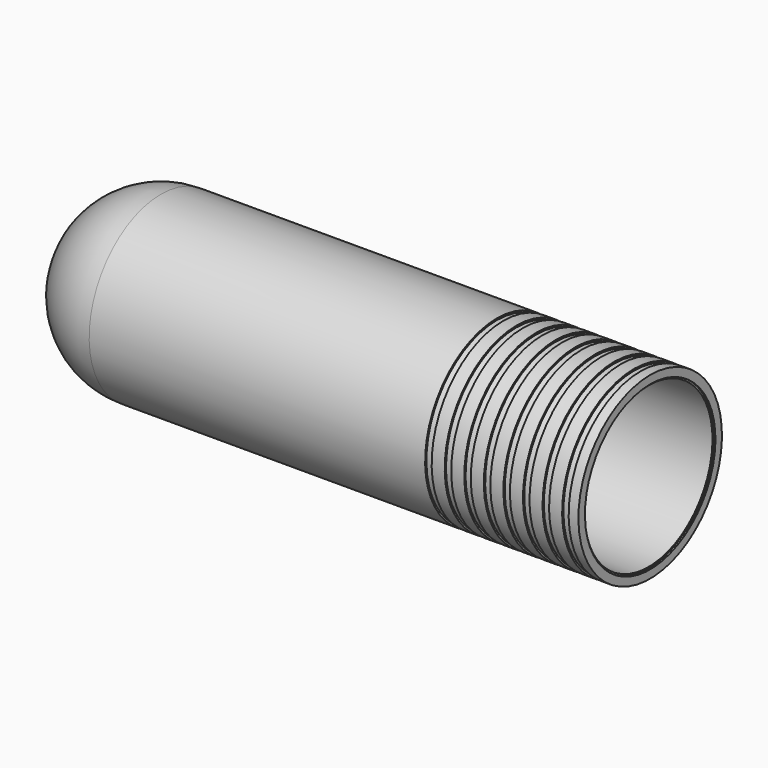
from build123d import *

# Parameters (mm, degrees)
F2_T = 2.5


# Not quite as in the source:
# - a shell that OpenCascade refuses in one call is made with other operations: the cavity is built on its own and cut out


with BuildPart() as f1:
    # F0 (on Front) → F1 (revolve)
    with BuildSketch(Plane.XZ):
        with BuildLine():
            Line((-96.4535274908, 0), (81.0464725092, 0))
            Line((81.0464725092, 0), (81.0464725092, 27.5))
            Line((81.0464725092, 27.5), (78.0464725092, 27.5))
            Line((78.0464725092, 27.5), (78.0464725092, 27))
            Line((78.0464725092, 27), (76.0464725092, 27))
            Line((76.0464725092, 27), (76.0464725092, 27.5))
            Line((76.0464725092, 27.5), (72.0464725092, 27.5))
            Line((72.0464725092, 27.5), (72.0464725092, 27))
            Line((72.0464725092, 27), (70.0464725092, 27))
            Line((70.0464725092, 27), (70.0464725092, 27.5))
            Line((70.0464725092, 27.5), (66.0464725092, 27.5))
            Line((66.0464725092, 27.5), (66.0464725092, 27))
            Line((66.0464725092, 27), (64.0464725092, 27))
            Line((64.0464725092, 27), (64.0464725092, 27.5))
            Line((64.0464725092, 27.5), (60.0464725092, 27.5))
            Line((60.0464725092, 27.5), (60.0464725092, 27))
            Line((60.0464725092, 27), (58.0464725092, 27))
            Line((58.0464725092, 27), (58.0464725092, 27.5))
            Line((58.0464725092, 27.5), (56.0464725092, 27.5))
            Line((56.0464725092, 27.5), (54.0464725092, 27.5))
            Line((54.0464725092, 27.5), (54.0464725092, 27))
            Line((54.0464725092, 27), (52.0464725092, 27))
            Line((52.0464725092, 27), (52.0464725092, 27.5))
            Line((52.0464725092, 27.5), (48.0464725092, 27.5))
            Line((48.0464725092, 27.5), (48.0464725092, 27))
            Line((48.0464725092, 27), (46.0464725092, 27))
            Line((46.0464725092, 27), (46.0464725092, 27.5))
            Line((46.0464725092, 27.5), (42.0464725092, 27.5))
            Line((42.0464725092, 27.5), (42.0464725092, 27))
            Line((42.0464725092, 27), (40.0464725092, 27))
            Line((40.0464725092, 27), (40.0464725092, 27.5))
            Line((40.0464725092, 27.5), (36.0464725092, 27.5))
            Line((36.0464725092, 27.5), (36.0464725092, 27))
            Line((36.0464725092, 27), (34.0464725092, 27))
            Line((34.0464725092, 27), (34.0464725092, 27.5))
            Line((34.0464725092, 27.5), (32.0464725092, 27.5))
            Line((32.0464725092, 27.5), (25.0464725092, 27.5))
            Line((25.0464725092, 27.5), (-68.9535274908, 27.5))
            ThreePointArc((-68.9535274908, 27.5), (-88.3989639735, 19.4454364826), (-96.4535274908, 0))
        make_face()
    revolve(axis=Axis((-7.7035274908, 0, 0), (-1, 0, 0)))

    # F2: shell of thickness 2.5, made by hand


with BuildPart() as f2_core1:
    # F2_t2: copy of F1
    add(f1.part)

    # the walls: a layer under each face that stays
    f2_faces = [f2_core1.faces().sort_by_distance(p)[0] for p in [
        (-88.3989639735, 0, -19.4454364826),
        (-17.4535274908, 0, -27.5),
        (34.0464725092, -13.2407407407, -24.0625),
        (35.0464725092, 0, -27),
        (36.0464725092, -13.2407407407, 24.0625),
        (38.0464725092, 0, -27.5),
        (40.0464725092, -13.2407407407, -24.0625),
        (41.0464725092, 0, -27),
        (42.0464725092, -13.2407407407, 24.0625),
        (44.0464725092, 0, -27.5),
        (46.0464725092, -13.2407407407, -24.0625),
        (47.0464725092, 0, -27),
        (48.0464725092, -13.2407407407, 24.0625),
        (50.0464725092, 0, -27.5),
        (52.0464725092, -13.2407407407, -24.0625),
        (53.0464725092, 0, -27),
        (54.0464725092, -13.2407407407, 24.0625),
        (56.0464725092, 0, -27.5),
        (58.0464725092, -13.2407407407, -24.0625),
        (59.0464725092, 0, -27),
        (60.0464725092, -13.2407407407, 24.0625),
        (62.0464725092, 0, -27.5),
        (64.0464725092, -13.2407407407, -24.0625),
        (65.0464725092, 0, -27),
        (66.0464725092, -13.2407407407, 24.0625),
        (68.0464725092, 0, -27.5),
        (70.0464725092, -13.2407407407, -24.0625),
        (71.0464725092, 0, -27),
        (72.0464725092, -13.2407407407, 24.0625),
        (74.0464725092, 0, -27.5),
        (76.0464725092, -13.2407407407, -24.0625),
        (77.0464725092, 0, -27),
        (78.0464725092, -13.2407407407, 24.0625),
        (79.5464725092, 0, -27.5),
    ]]
    thicken(f2_faces, amount=-F2_T, mode=Mode.SUBTRACT)

    # F2_s3 → F2_t4 (revolve, cut)
    with BuildSketch(Plane.XZ):
        Polygon((34.0714725092, 27.025), (31.5464725092, 27), (31.5464725092, 24.5), (34.0464725092, 24.5), align=None)
    revolve(axis=Axis((34.0464725092, 0, 0), (-1, 0, 0)), mode=Mode.SUBTRACT)

    # F2_s5 → F2_t6 (revolve, cut)
    with BuildSketch(Plane.XZ):
        Polygon((36.0214725092, 27.025), (36.0464725092, 24.5), (38.5464725092, 24.5), (38.5464725092, 27), align=None)
    revolve(axis=Axis((36.0464725092, 0, 0), (-1, 0, 0)), mode=Mode.SUBTRACT)

    # F2_s7 → F2_t8 (revolve, cut)
    with BuildSketch(Plane.XZ):
        Polygon((40.0714725092, 27.025), (37.5464725092, 27), (37.5464725092, 24.5), (40.0464725092, 24.5), align=None)
    revolve(axis=Axis((40.0464725092, 0, 0), (-1, 0, 0)), mode=Mode.SUBTRACT)

    # F2_s9 → F2_t10 (revolve, cut)
    with BuildSketch(Plane.XZ):
        Polygon((42.0214725092, 27.025), (42.0464725092, 24.5), (44.5464725092, 24.5), (44.5464725092, 27), align=None)
    revolve(axis=Axis((42.0464725092, 0, 0), (-1, 0, 0)), mode=Mode.SUBTRACT)

    # F2_s11 → F2_t12 (revolve, cut)
    with BuildSketch(Plane.XZ):
        Polygon((46.0714725092, 27.025), (43.5464725092, 27), (43.5464725092, 24.5), (46.0464725092, 24.5), align=None)
    revolve(axis=Axis((46.0464725092, 0, 0), (-1, 0, 0)), mode=Mode.SUBTRACT)

    # F2_s13 → F2_t14 (revolve, cut)
    with BuildSketch(Plane.XZ):
        Polygon((48.0214725092, 27.025), (48.0464725092, 24.5), (50.5464725092, 24.5), (50.5464725092, 27), align=None)
    revolve(axis=Axis((48.0464725092, 0, 0), (-1, 0, 0)), mode=Mode.SUBTRACT)

    # F2_s15 → F2_t16 (revolve, cut)
    with BuildSketch(Plane.XZ):
        Polygon((52.0714725092, 27.025), (49.5464725092, 27), (49.5464725092, 24.5), (52.0464725092, 24.5), align=None)
    revolve(axis=Axis((52.0464725092, 0, 0), (-1, 0, 0)), mode=Mode.SUBTRACT)

    # F2_s17 → F2_t18 (revolve, cut)
    with BuildSketch(Plane.XZ):
        Polygon((54.0214725092, 27.025), (54.0464725092, 24.5), (56.5464725092, 24.5), (56.5464725092, 27), align=None)
    revolve(axis=Axis((54.0464725092, 0, 0), (-1, 0, 0)), mode=Mode.SUBTRACT)

    # F2_s19 → F2_t20 (revolve, cut)
    with BuildSketch(Plane.XZ):
        Polygon((58.0714725092, 27.025), (55.5464725092, 27), (55.5464725092, 24.5), (58.0464725092, 24.5), align=None)
    revolve(axis=Axis((58.0464725092, 0, 0), (-1, 0, 0)), mode=Mode.SUBTRACT)

    # F2_s21 → F2_t22 (revolve, cut)
    with BuildSketch(Plane.XZ):
        Polygon((60.0214725092, 27.025), (60.0464725092, 24.5), (62.5464725092, 24.5), (62.5464725092, 27), align=None)
    revolve(axis=Axis((60.0464725092, 0, 0), (-1, 0, 0)), mode=Mode.SUBTRACT)

    # F2_s23 → F2_t24 (revolve, cut)
    with BuildSketch(Plane.XZ):
        Polygon((64.0714725092, 27.025), (61.5464725092, 27), (61.5464725092, 24.5), (64.0464725092, 24.5), align=None)
    revolve(axis=Axis((64.0464725092, 0, 0), (-1, 0, 0)), mode=Mode.SUBTRACT)

    # F2_s25 → F2_t26 (revolve, cut)
    with BuildSketch(Plane.XZ):
        Polygon((66.0214725092, 27.025), (66.0464725092, 24.5), (68.5464725092, 24.5), (68.5464725092, 27), align=None)
    revolve(axis=Axis((66.0464725092, 0, 0), (-1, 0, 0)), mode=Mode.SUBTRACT)

    # F2_s27 → F2_t28 (revolve, cut)
    with BuildSketch(Plane.XZ):
        Polygon((70.0714725092, 27.025), (67.5464725092, 27), (67.5464725092, 24.5), (70.0464725092, 24.5), align=None)
    revolve(axis=Axis((70.0464725092, 0, 0), (-1, 0, 0)), mode=Mode.SUBTRACT)

    # F2_s29 → F2_t30 (revolve, cut)
    with BuildSketch(Plane.XZ):
        Polygon((72.0214725092, 27.025), (72.0464725092, 24.5), (74.5464725092, 24.5), (74.5464725092, 27), align=None)
    revolve(axis=Axis((72.0464725092, 0, 0), (-1, 0, 0)), mode=Mode.SUBTRACT)

    # F2_s31 → F2_t32 (revolve, cut)
    with BuildSketch(Plane.XZ):
        Polygon((76.0714725092, 27.025), (73.5464725092, 27), (73.5464725092, 24.5), (76.0464725092, 24.5), align=None)
    revolve(axis=Axis((76.0464725092, 0, 0), (-1, 0, 0)), mode=Mode.SUBTRACT)

    # F2_s33 → F2_t34 (revolve, cut)
    with BuildSketch(Plane.XZ):
        Polygon((78.0214725092, 27.025), (78.0464725092, 24.5), (80.5464725092, 24.5), (80.5464725092, 27), align=None)
    revolve(axis=Axis((78.0464725092, 0, 0), (-1, 0, 0)), mode=Mode.SUBTRACT)


with BuildPart() as f1_1:
    add(f1.part)

    # what is left inside the walls is the cavity
    f2_cavity = [f2_core1.part.solids().sort_by_distance(p)[0] for p in [
        (-1.953527, 0, -24.975),
    ]]
    add(f2_cavity, mode=Mode.SUBTRACT)


solid = f1_1.part
